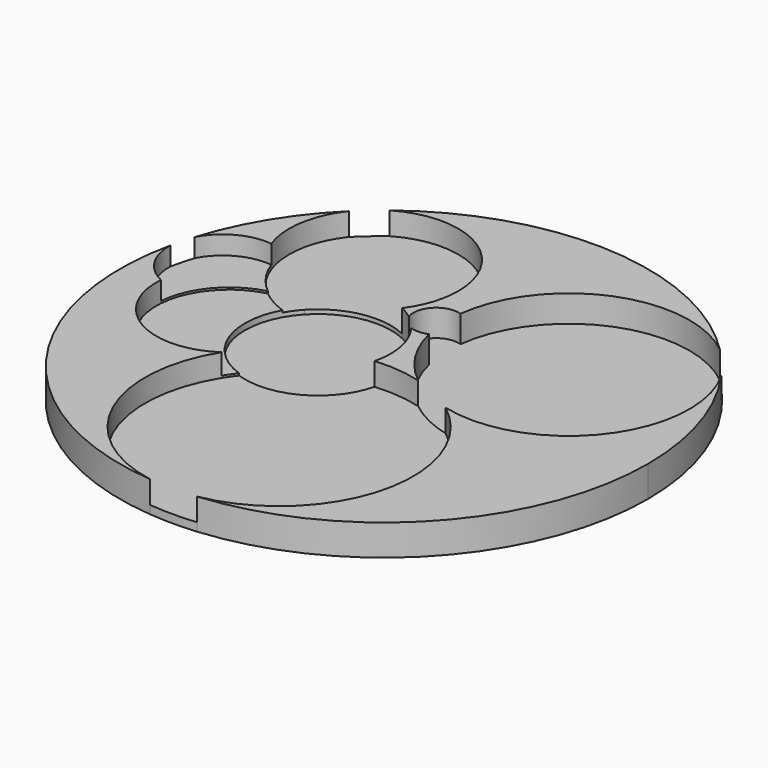
from build123d import *

# Parameters (mm, degrees)
F1_DEPTH = 1.5
F2_DEPTH = 1.1
F3_DEPTH = 1.3
F4_DEPTH = 1
F5_DEPTH = 0.9
F6_DEPTH = 1.3
F7_DEPTH = 1.3
F8_DEPTH = 1.1


with BuildPart() as f1:
    # F0 (on Top) → F1 (new body)
    with BuildSketch(Plane.XY):
        with BuildLine():
            ThreePointArc((1.1413139167, -12.749015748), (9.4458673009, -8.6380316585), (12.8, 0))
            ThreePointArc((12.8, 0), (12.2037895541, 3.8610258375), (10.470699919, 7.3623666851))
            ThreePointArc((10.470699919, 7.3623666851), (10.0212563072, 0.9384212672), (3.9401496855, -1.1803558676))
            ThreePointArc((3.9401496855, -1.1803558676), (6.3177362198, -7.8784662435), (1.1413139167, -12.749015748))
        make_face()
        with BuildLine():
            ThreePointArc((3.9401496855, -1.1803558676), (10.0212563072, 0.9384212672), (10.470699919, 7.3623666851))
            ThreePointArc((10.470699919, 7.3623666851), (9.8213681495, 8.2085764705), (9.1038369322, 8.9977860117))
            ThreePointArc((9.1038369322, 8.9977860117), (3.2034297018, 9.9238080984), (-0.4347578085, 5.1871516796))
            ThreePointArc((-0.4347578085, 5.1871516796), (0.1140807918, 4.7873856476), (0.3236429235, 4.1415370565))
            ThreePointArc((0.3236429235, 4.1415370565), (0.1493131035, 3.5472856637), (-0.3184201999, 3.1413901588))
            ThreePointArc((-0.3184201999, 3.1413901588), (0.4342128527, 1.3569660974), (1.7281912806, -0.0839522107))
            ThreePointArc((1.7281912806, -0.0839522107), (2.8867018502, -0.5261737296), (3.9401496855, -1.1803558676))
        make_face()
        with BuildLine():
            ThreePointArc((-1.1413139167, -12.749015748), (0, -12.8), (1.1413139167, -12.749015748))
            ThreePointArc((1.1413139167, -12.749015748), (6.3177362198, -7.8784662435), (3.9401496855, -1.1803558676))
            ThreePointArc((3.9401496855, -1.1803558676), (2.7756748559, -0.7501670477), (1.7281912806, -0.0839522107))
            ThreePointArc((1.7281912806, -0.0839522107), (0.596280043, 0.1225922249), (-0.554315346, 0.1263210619))
            ThreePointArc((-0.554315346, 0.1263210619), (-2.2047100942, -2.0697503993), (-4.9291383896, -2.4219196064))
            ThreePointArc((-4.9291383896, -2.4219196064), (-5.2141366822, -2.6925550862), (-5.5274388721, -2.9298509512))
            ThreePointArc((-5.5274388721, -2.9298509512), (-5.9348180483, -9.0010252232), (-1.1413139167, -12.749015748))
        make_face()
        with BuildLine():
            ThreePointArc((-0.4347578085, 5.1871516796), (3.2034297018, 9.9238080984), (9.1038369322, 8.9977860117))
            ThreePointArc((9.1038369322, 8.9977860117), (0.8515670805, 12.7716417702), (-7.8286793929, 10.1267852235))
            ThreePointArc((-7.8286793929, 10.1267852235), (-3.7190007865, 10.1436555147), (-1.6592760481, 6.5873545071))
            ThreePointArc((-1.6592760481, 6.5873545071), (-1.8611994375, 5.316528501), (-2.4470803104, 4.1708778581))
            ThreePointArc((-2.4470803104, 4.1708778581), (-2.1205912314, 3.9914565549), (-1.8147879972, 3.7786855401))
            ThreePointArc((-1.8147879972, 3.7786855401), (-1.5620655496, 4.9113826225), (-0.4347578085, 5.1871516796))
        make_face()
        with BuildLine():
            ThreePointArc((1.7281912806, -0.0839522107), (2.7756748559, -0.7501670477), (3.9401496855, -1.1803558676))
            ThreePointArc((3.9401496855, -1.1803558676), (2.8867018502, -0.5261737296), (1.7281912806, -0.0839522107))
        make_face()
        with BuildLine():
            ThreePointArc((-12.5092777133, 2.7125580349), (-10.3126004927, -7.5822339107), (-1.1413139167, -12.749015748))
            ThreePointArc((-1.1413139167, -12.749015748), (-5.9348180483, -9.0010252232), (-5.5274388721, -2.9298509512))
            ThreePointArc((-5.5274388721, -2.9298509512), (-9.2745377761, -3.053856526), (-11.0221912783, 0.2630448617))
            ThreePointArc((-11.0221912783, 0.2630448617), (-12.1336526301, 1.2644403034), (-12.5092777133, 2.7125580349))
        make_face()
        with BuildLine():
            ThreePointArc((-1.6592760481, 6.5873545071), (-3.7190007865, 10.1436555147), (-7.8286793929, 10.1267852235))
            ThreePointArc((-7.8286793929, 10.1267852235), (-8.4249981047, 9.6363585932), (-8.9906633635, 9.1108711046))
            ThreePointArc((-8.9906633635, 9.1108711046), (-9.8078763851, 7.234529376), (-9.6163122558, 5.1969330987))
            ThreePointArc((-9.6163122558, 5.1969330987), (-8.3134717361, 4.6648999744), (-7.4786994453, 3.5319357704))
            ThreePointArc((-7.4786994453, 3.5319357704), (-7.0171820767, 3.4988442167), (-6.5639507121, 3.4057063483))
            ThreePointArc((-6.5639507121, 3.4057063483), (-4.6309358982, 4.4630943822), (-2.4470803104, 4.1708778581))
            ThreePointArc((-2.4470803104, 4.1708778581), (-1.8611994375, 5.316528501), (-1.6592760481, 6.5873545071))
        make_face()
        with BuildLine():
            ThreePointArc((0.3236429235, 4.1415370565), (0.1140807918, 4.7873856476), (-0.4347578085, 5.1871516796))
            ThreePointArc((-0.4347578085, 5.1871516796), (-0.4668571228, 4.1591375853), (-0.3184201999, 3.1413901588))
            ThreePointArc((-0.3184201999, 3.1413901588), (0.1493131035, 3.5472856637), (0.3236429235, 4.1415370565))
        make_face()
        with BuildLine():
            ThreePointArc((-0.3184201999, 3.1413901588), (-0.4668571228, 4.1591375853), (-0.4347578085, 5.1871516796))
            ThreePointArc((-0.4347578085, 5.1871516796), (-1.5620655496, 4.9113826225), (-1.8147879972, 3.7786855401))
            ThreePointArc((-1.8147879972, 3.7786855401), (-1.4632990979, 3.4659314694), (-1.1564367138, 3.1092873438))
            ThreePointArc((-1.1564367138, 3.1092873438), (-0.7342490593, 3.0423432998), (-0.3184201999, 3.1413901588))
        make_face()
        with BuildLine():
            ThreePointArc((-0.554315346, 0.1263210619), (0.596280043, 0.1225922249), (1.7281912806, -0.0839522107))
            ThreePointArc((1.7281912806, -0.0839522107), (0.4342128527, 1.3569660974), (-0.3184201999, 3.1413901588))
            ThreePointArc((-0.3184201999, 3.1413901588), (-0.7342490593, 3.0423432998), (-1.1564367138, 3.1092873438))
            ThreePointArc((-1.1564367138, 3.1092873438), (-0.6299288982, 2.1052191407), (-0.4482007155, 0.9861399191))
            ThreePointArc((-0.4482007155, 0.9861399191), (-0.4748296274, 0.5529688265), (-0.554315346, 0.1263210619))
        make_face()
        with BuildLine():
            ThreePointArc((-12.2201512567, 3.8089241608), (-12.3768602224, 3.2639440918), (-12.5092777133, 2.7125580349))
            ThreePointArc((-12.5092777133, 2.7125580349), (-12.1336526301, 1.2644403034), (-11.0221912783, 0.2630448617))
            ThreePointArc((-11.0221912783, 0.2630448617), (-10.204575831, 2.2716279569), (-8.3673749649, 3.4238406316))
            ThreePointArc((-8.3673749649, 3.4238406316), (-9.1112094109, 4.2263075504), (-9.6163122558, 5.1969330987))
            ThreePointArc((-9.6163122558, 5.1969330987), (-11.1342032079, 4.90808084), (-12.2201512567, 3.8089241608))
        make_face()
        with BuildLine():
            ThreePointArc((-11.0221912783, 0.2630448617), (-9.2745377761, -3.053856526), (-5.5274388721, -2.9298509512))
            ThreePointArc((-5.5274388721, -2.9298509512), (-5.3367748168, -2.6393619746), (-5.1308600113, -2.3594767831))
            ThreePointArc((-5.1308600113, -2.3594767831), (-7.2860930404, -0.2817879048), (-7.075700244, 2.704439708))
            ThreePointArc((-7.075700244, 2.704439708), (-7.1973059974, 2.7478141876), (-7.3174857567, 2.7949960715))
            ThreePointArc((-7.3174857567, 2.7949960715), (-8.4441033358, 0.4671377871), (-11.0221912783, 0.2630448617))
        make_face()
        with BuildLine():
            ThreePointArc((-5.1308600113, -2.3594767831), (-5.3367748168, -2.6393619746), (-5.5274388721, -2.9298509512))
            ThreePointArc((-5.5274388721, -2.9298509512), (-5.2141366822, -2.6925550862), (-4.9291383896, -2.4219196064))
            ThreePointArc((-4.9291383896, -2.4219196064), (-5.0304653636, -2.3922041354), (-5.1308600113, -2.3594767831))
        make_face()
        with BuildLine():
            ThreePointArc((-9.6163122558, 5.1969330987), (-9.8078763851, 7.234529376), (-8.9906633635, 9.1108711046))
            ThreePointArc((-8.9906633635, 9.1108711046), (-10.931711877, 6.6586541762), (-12.2201512567, 3.8089241608))
            ThreePointArc((-12.2201512567, 3.8089241608), (-11.1342032079, 4.90808084), (-9.6163122558, 5.1969330987))
        make_face()
        with BuildLine():
            ThreePointArc((-1.1564367138, 3.1092873438), (-1.5606188549, 3.3702177563), (-1.8147879972, 3.7786855401))
            ThreePointArc((-1.8147879972, 3.7786855401), (-2.1205912314, 3.9914565549), (-2.4470803104, 4.1708778581))
            ThreePointArc((-2.4470803104, 4.1708778581), (-3.5931195136, 3.1062963536), (-5.0544484876, 2.5483920029))
            ThreePointArc((-5.0544484876, 2.5483920029), (-4.2509453728, 1.3851599291), (-3.968, 0))
            ThreePointArc((-3.968, 0), (-4.048144568, -0.7481430857), (-4.2849411533, -1.4623339606))
            ThreePointArc((-4.2849411533, -1.4623339606), (-2.5466756884, -0.3696619712), (-0.554315346, 0.1263210619))
            ThreePointArc((-0.554315346, 0.1263210619), (-0.4748296274, 0.5529688265), (-0.4482007155, 0.9861399191))
            ThreePointArc((-0.4482007155, 0.9861399191), (-0.6299288982, 2.1052191407), (-1.1564367138, 3.1092873438))
        make_face()
        with BuildLine():
            ThreePointArc((-1.1564367138, 3.1092873438), (-1.4632990979, 3.4659314694), (-1.8147879972, 3.7786855401))
            ThreePointArc((-1.8147879972, 3.7786855401), (-1.5606188549, 3.3702177563), (-1.1564367138, 3.1092873438))
        make_face()
        with BuildLine():
            ThreePointArc((-4.9291383896, -2.4219196064), (-2.2047100942, -2.0697503993), (-0.554315346, 0.1263210619))
            ThreePointArc((-0.554315346, 0.1263210619), (-2.5466756884, -0.3696619712), (-4.2849411533, -1.4623339606))
            ThreePointArc((-4.2849411533, -1.4623339606), (-4.5675232248, -1.9686553693), (-4.9291383896, -2.4219196064))
        make_face()
        with BuildLine():
            ThreePointArc((-8.3673749649, 3.4238406316), (-10.204575831, 2.2716279569), (-11.0221912783, 0.2630448617))
            ThreePointArc((-11.0221912783, 0.2630448617), (-8.4441033358, 0.4671377871), (-7.3174857567, 2.7949960715))
            ThreePointArc((-7.3174857567, 2.7949960715), (-7.8660255018, 3.0700250173), (-8.3673749649, 3.4238406316))
        make_face()
        with BuildLine():
            ThreePointArc((-7.075700244, 2.704439708), (-7.2860930404, -0.2817879048), (-5.1308600113, -2.3594767831))
            ThreePointArc((-5.1308600113, -2.3594767831), (-4.7292223678, -1.8908009917), (-4.2849411533, -1.4623339606))
            ThreePointArc((-4.2849411533, -1.4623339606), (-4.048144568, -0.7481430857), (-3.968, 0))
            ThreePointArc((-3.968, 0), (-4.2509453728, 1.3851599291), (-5.0544484876, 2.5483920029))
            ThreePointArc((-5.0544484876, 2.5483920029), (-6.0748712519, 2.4995189346), (-7.075700244, 2.704439708))
        make_face()
        with BuildLine():
            ThreePointArc((-4.2849411533, -1.4623339606), (-4.7292223678, -1.8908009917), (-5.1308600113, -2.3594767831))
            ThreePointArc((-5.1308600113, -2.3594767831), (-5.0304653636, -2.3922041354), (-4.9291383896, -2.4219196064))
            ThreePointArc((-4.9291383896, -2.4219196064), (-4.5675232248, -1.9686553693), (-4.2849411533, -1.4623339606))
        make_face()
        with BuildLine():
            ThreePointArc((-7.4786994453, 3.5319357704), (-8.3134717361, 4.6648999744), (-9.6163122558, 5.1969330987))
            ThreePointArc((-9.6163122558, 5.1969330987), (-9.1112094109, 4.2263075504), (-8.3673749649, 3.4238406316))
            ThreePointArc((-8.3673749649, 3.4238406316), (-7.9264758102, 3.5061577807), (-7.4786994453, 3.5319357704))
        make_face()
        with BuildLine():
            ThreePointArc((-5.0544484876, 2.5483920029), (-3.5931195136, 3.1062963536), (-2.4470803104, 4.1708778581))
            ThreePointArc((-2.4470803104, 4.1708778581), (-4.6309358982, 4.4630943822), (-6.5639507121, 3.4057063483))
            ThreePointArc((-6.5639507121, 3.4057063483), (-5.7557084634, 3.0712328201), (-5.0544484876, 2.5483920029))
        make_face()
        with BuildLine():
            ThreePointArc((-7.4786994453, 3.5319357704), (-7.9264758102, 3.5061577807), (-8.3673749649, 3.4238406316))
            ThreePointArc((-8.3673749649, 3.4238406316), (-7.8660255018, 3.0700250173), (-7.3174857567, 2.7949960715))
            ThreePointArc((-7.3174857567, 2.7949960715), (-7.3712234042, 3.1693438542), (-7.4786994453, 3.5319357704))
        make_face()
        with BuildLine():
            ThreePointArc((-7.4786994453, 3.5319357704), (-7.3712234042, 3.1693438542), (-7.3174857567, 2.7949960715))
            ThreePointArc((-7.3174857567, 2.7949960715), (-7.1973059974, 2.7478141876), (-7.075700244, 2.704439708))
            ThreePointArc((-7.075700244, 2.704439708), (-6.8414254387, 3.0708356057), (-6.5639507121, 3.4057063483))
            ThreePointArc((-6.5639507121, 3.4057063483), (-7.0171820767, 3.4988442167), (-7.4786994453, 3.5319357704))
        make_face()
        with BuildLine():
            ThreePointArc((-6.5639507121, 3.4057063483), (-6.8414254387, 3.0708356057), (-7.075700244, 2.704439708))
            ThreePointArc((-7.075700244, 2.704439708), (-6.0748712519, 2.4995189346), (-5.0544484876, 2.5483920029))
            ThreePointArc((-5.0544484876, 2.5483920029), (-5.7557084634, 3.0712328201), (-6.5639507121, 3.4057063483))
        make_face()
    extrude(amount=-F1_DEPTH)

    # F0 (on Top) → F2 (cut)
    with BuildSketch(Plane.XY):
        with BuildLine():
            ThreePointArc((-1.1413139167, -12.749015748), (0, -12.85), (1.1413139167, -12.749015748))
            ThreePointArc((1.1413139167, -12.749015748), (0, -12.8), (-1.1413139167, -12.749015748))
        make_face()
        with BuildLine():
            ThreePointArc((-1.1413139167, -12.749015748), (0, -12.8), (1.1413139167, -12.749015748))
            ThreePointArc((1.1413139167, -12.749015748), (6.3177362198, -7.8784662435), (3.9401496855, -1.1803558676))
            ThreePointArc((3.9401496855, -1.1803558676), (2.7756748559, -0.7501670477), (1.7281912806, -0.0839522107))
            ThreePointArc((1.7281912806, -0.0839522107), (0.596280043, 0.1225922249), (-0.554315346, 0.1263210619))
            ThreePointArc((-0.554315346, 0.1263210619), (-2.2047100942, -2.0697503993), (-4.9291383896, -2.4219196064))
            ThreePointArc((-4.9291383896, -2.4219196064), (-5.2141366822, -2.6925550862), (-5.5274388721, -2.9298509512))
            ThreePointArc((-5.5274388721, -2.9298509512), (-5.9348180483, -9.0010252232), (-1.1413139167, -12.749015748))
        make_face()
        with BuildLine():
            ThreePointArc((1.7281912806, -0.0839522107), (2.7756748559, -0.7501670477), (3.9401496855, -1.1803558676))
            ThreePointArc((3.9401496855, -1.1803558676), (2.8867018502, -0.5261737296), (1.7281912806, -0.0839522107))
        make_face()
        with BuildLine():
            ThreePointArc((-4.9291383896, -2.4219196064), (-2.2047100942, -2.0697503993), (-0.554315346, 0.1263210619))
            ThreePointArc((-0.554315346, 0.1263210619), (-2.5466756884, -0.3696619712), (-4.2849411533, -1.4623339606))
            ThreePointArc((-4.2849411533, -1.4623339606), (-4.5675232248, -1.9686553693), (-4.9291383896, -2.4219196064))
        make_face()
        with BuildLine():
            ThreePointArc((-4.2849411533, -1.4623339606), (-4.7292223678, -1.8908009917), (-5.1308600113, -2.3594767831))
            ThreePointArc((-5.1308600113, -2.3594767831), (-5.0304653636, -2.3922041354), (-4.9291383896, -2.4219196064))
            ThreePointArc((-4.9291383896, -2.4219196064), (-4.5675232248, -1.9686553693), (-4.2849411533, -1.4623339606))
        make_face()
        with BuildLine():
            ThreePointArc((-5.1308600113, -2.3594767831), (-5.3367748168, -2.6393619746), (-5.5274388721, -2.9298509512))
            ThreePointArc((-5.5274388721, -2.9298509512), (-5.2141366822, -2.6925550862), (-4.9291383896, -2.4219196064))
            ThreePointArc((-4.9291383896, -2.4219196064), (-5.0304653636, -2.3922041354), (-5.1308600113, -2.3594767831))
        make_face()
    extrude(amount=-F2_DEPTH, mode=Mode.SUBTRACT)

    # F0 (on Top) → F3 (cut)
    with BuildSketch(Plane.XY):
        with BuildLine():
            ThreePointArc((-7.075700244, 2.704439708), (-7.2860930404, -0.2817879048), (-5.1308600113, -2.3594767831))
            ThreePointArc((-5.1308600113, -2.3594767831), (-4.7292223678, -1.8908009917), (-4.2849411533, -1.4623339606))
            ThreePointArc((-4.2849411533, -1.4623339606), (-4.048144568, -0.7481430857), (-3.968, 0))
            ThreePointArc((-3.968, 0), (-4.2509453728, 1.3851599291), (-5.0544484876, 2.5483920029))
            ThreePointArc((-5.0544484876, 2.5483920029), (-6.0748712519, 2.4995189346), (-7.075700244, 2.704439708))
        make_face()
        with BuildLine():
            ThreePointArc((-1.1564367138, 3.1092873438), (-1.5606188549, 3.3702177563), (-1.8147879972, 3.7786855401))
            ThreePointArc((-1.8147879972, 3.7786855401), (-2.1205912314, 3.9914565549), (-2.4470803104, 4.1708778581))
            ThreePointArc((-2.4470803104, 4.1708778581), (-3.5931195136, 3.1062963536), (-5.0544484876, 2.5483920029))
            ThreePointArc((-5.0544484876, 2.5483920029), (-4.2509453728, 1.3851599291), (-3.968, 0))
            ThreePointArc((-3.968, 0), (-4.048144568, -0.7481430857), (-4.2849411533, -1.4623339606))
            ThreePointArc((-4.2849411533, -1.4623339606), (-2.5466756884, -0.3696619712), (-0.554315346, 0.1263210619))
            ThreePointArc((-0.554315346, 0.1263210619), (-0.4748296274, 0.5529688265), (-0.4482007155, 0.9861399191))
            ThreePointArc((-0.4482007155, 0.9861399191), (-0.6299288982, 2.1052191407), (-1.1564367138, 3.1092873438))
        make_face()
        with BuildLine():
            ThreePointArc((-5.0544484876, 2.5483920029), (-3.5931195136, 3.1062963536), (-2.4470803104, 4.1708778581))
            ThreePointArc((-2.4470803104, 4.1708778581), (-4.6309358982, 4.4630943822), (-6.5639507121, 3.4057063483))
            ThreePointArc((-6.5639507121, 3.4057063483), (-5.7557084634, 3.0712328201), (-5.0544484876, 2.5483920029))
        make_face()
        with BuildLine():
            ThreePointArc((-6.5639507121, 3.4057063483), (-6.8414254387, 3.0708356057), (-7.075700244, 2.704439708))
            ThreePointArc((-7.075700244, 2.704439708), (-6.0748712519, 2.4995189346), (-5.0544484876, 2.5483920029))
            ThreePointArc((-5.0544484876, 2.5483920029), (-5.7557084634, 3.0712328201), (-6.5639507121, 3.4057063483))
        make_face()
        with BuildLine():
            ThreePointArc((-4.9291383896, -2.4219196064), (-2.2047100942, -2.0697503993), (-0.554315346, 0.1263210619))
            ThreePointArc((-0.554315346, 0.1263210619), (-2.5466756884, -0.3696619712), (-4.2849411533, -1.4623339606))
            ThreePointArc((-4.2849411533, -1.4623339606), (-4.5675232248, -1.9686553693), (-4.9291383896, -2.4219196064))
        make_face()
        with BuildLine():
            ThreePointArc((-4.2849411533, -1.4623339606), (-4.7292223678, -1.8908009917), (-5.1308600113, -2.3594767831))
            ThreePointArc((-5.1308600113, -2.3594767831), (-5.0304653636, -2.3922041354), (-4.9291383896, -2.4219196064))
            ThreePointArc((-4.9291383896, -2.4219196064), (-4.5675232248, -1.9686553693), (-4.2849411533, -1.4623339606))
        make_face()
        with BuildLine():
            ThreePointArc((-1.1564367138, 3.1092873438), (-1.4632990979, 3.4659314694), (-1.8147879972, 3.7786855401))
            ThreePointArc((-1.8147879972, 3.7786855401), (-1.5606188549, 3.3702177563), (-1.1564367138, 3.1092873438))
        make_face()
    extrude(amount=-F3_DEPTH, mode=Mode.SUBTRACT)

    # F0 (on Top) → F4 (cut)
    with BuildSketch(Plane.XY):
        with BuildLine():
            ThreePointArc((-11.0221912783, 0.2630448617), (-9.2745377761, -3.053856526), (-5.5274388721, -2.9298509512))
            ThreePointArc((-5.5274388721, -2.9298509512), (-5.3367748168, -2.6393619746), (-5.1308600113, -2.3594767831))
            ThreePointArc((-5.1308600113, -2.3594767831), (-7.2860930404, -0.2817879048), (-7.075700244, 2.704439708))
            ThreePointArc((-7.075700244, 2.704439708), (-7.1973059974, 2.7478141876), (-7.3174857567, 2.7949960715))
            ThreePointArc((-7.3174857567, 2.7949960715), (-8.4441033358, 0.4671377871), (-11.0221912783, 0.2630448617))
        make_face()
        with BuildLine():
            ThreePointArc((-8.3673749649, 3.4238406316), (-10.204575831, 2.2716279569), (-11.0221912783, 0.2630448617))
            ThreePointArc((-11.0221912783, 0.2630448617), (-8.4441033358, 0.4671377871), (-7.3174857567, 2.7949960715))
            ThreePointArc((-7.3174857567, 2.7949960715), (-7.8660255018, 3.0700250173), (-8.3673749649, 3.4238406316))
        make_face()
        with BuildLine():
            ThreePointArc((-7.4786994453, 3.5319357704), (-7.9264758102, 3.5061577807), (-8.3673749649, 3.4238406316))
            ThreePointArc((-8.3673749649, 3.4238406316), (-7.8660255018, 3.0700250173), (-7.3174857567, 2.7949960715))
            ThreePointArc((-7.3174857567, 2.7949960715), (-7.3712234042, 3.1693438542), (-7.4786994453, 3.5319357704))
        make_face()
        with BuildLine():
            ThreePointArc((-7.4786994453, 3.5319357704), (-7.3712234042, 3.1693438542), (-7.3174857567, 2.7949960715))
            ThreePointArc((-7.3174857567, 2.7949960715), (-7.1973059974, 2.7478141876), (-7.075700244, 2.704439708))
            ThreePointArc((-7.075700244, 2.704439708), (-6.8414254387, 3.0708356057), (-6.5639507121, 3.4057063483))
            ThreePointArc((-6.5639507121, 3.4057063483), (-7.0171820767, 3.4988442167), (-7.4786994453, 3.5319357704))
        make_face()
    extrude(amount=-F4_DEPTH, mode=Mode.SUBTRACT)

    # F0 (on Top) → F5 (cut)
    with BuildSketch(Plane.XY):
        with BuildLine():
            ThreePointArc((-12.2201512567, 3.8089241608), (-12.3768602224, 3.2639440918), (-12.5092777133, 2.7125580349))
            ThreePointArc((-12.5092777133, 2.7125580349), (-12.1336526301, 1.2644403034), (-11.0221912783, 0.2630448617))
            ThreePointArc((-11.0221912783, 0.2630448617), (-10.204575831, 2.2716279569), (-8.3673749649, 3.4238406316))
            ThreePointArc((-8.3673749649, 3.4238406316), (-9.1112094109, 4.2263075504), (-9.6163122558, 5.1969330987))
            ThreePointArc((-9.6163122558, 5.1969330987), (-11.1342032079, 4.90808084), (-12.2201512567, 3.8089241608))
        make_face()
        with BuildLine():
            ThreePointArc((-7.4786994453, 3.5319357704), (-8.3134717361, 4.6648999744), (-9.6163122558, 5.1969330987))
            ThreePointArc((-9.6163122558, 5.1969330987), (-9.1112094109, 4.2263075504), (-8.3673749649, 3.4238406316))
            ThreePointArc((-8.3673749649, 3.4238406316), (-7.9264758102, 3.5061577807), (-7.4786994453, 3.5319357704))
        make_face()
    extrude(amount=-F5_DEPTH, mode=Mode.SUBTRACT)

    # F0 (on Top) → F6 (cut)
    with BuildSketch(Plane.XY):
        with BuildLine():
            ThreePointArc((3.9401496855, -1.1803558676), (10.0212563072, 0.9384212672), (10.470699919, 7.3623666851))
            ThreePointArc((10.470699919, 7.3623666851), (9.8213681495, 8.2085764705), (9.1038369322, 8.9977860117))
            ThreePointArc((9.1038369322, 8.9977860117), (3.2034297018, 9.9238080984), (-0.4347578085, 5.1871516796))
            ThreePointArc((-0.4347578085, 5.1871516796), (0.1140807918, 4.7873856476), (0.3236429235, 4.1415370565))
            ThreePointArc((0.3236429235, 4.1415370565), (0.1493131035, 3.5472856637), (-0.3184201999, 3.1413901588))
            ThreePointArc((-0.3184201999, 3.1413901588), (0.4342128527, 1.3569660974), (1.7281912806, -0.0839522107))
            ThreePointArc((1.7281912806, -0.0839522107), (2.8867018502, -0.5261737296), (3.9401496855, -1.1803558676))
        make_face()
        with BuildLine():
            ThreePointArc((0.3236429235, 4.1415370565), (0.1140807918, 4.7873856476), (-0.4347578085, 5.1871516796))
            ThreePointArc((-0.4347578085, 5.1871516796), (-0.4668571228, 4.1591375853), (-0.3184201999, 3.1413901588))
            ThreePointArc((-0.3184201999, 3.1413901588), (0.1493131035, 3.5472856637), (0.3236429235, 4.1415370565))
        make_face()
        with BuildLine():
            ThreePointArc((1.7281912806, -0.0839522107), (2.7756748559, -0.7501670477), (3.9401496855, -1.1803558676))
            ThreePointArc((3.9401496855, -1.1803558676), (2.8867018502, -0.5261737296), (1.7281912806, -0.0839522107))
        make_face()
        with BuildLine():
            ThreePointArc((9.1038369322, 8.9977860117), (9.8213681495, 8.2085764705), (10.470699919, 7.3623666851))
            ThreePointArc((10.470699919, 7.3623666851), (9.8623786831, 8.2428525608), (9.1038369322, 8.9977860117))
        make_face()
    extrude(amount=-F6_DEPTH, mode=Mode.SUBTRACT)

    # F0 (on Top) → F7 (cut)
    with BuildSketch(Plane.XY):
        with BuildLine():
            ThreePointArc((-0.3184201999, 3.1413901588), (-0.4668571228, 4.1591375853), (-0.4347578085, 5.1871516796))
            ThreePointArc((-0.4347578085, 5.1871516796), (-1.5620655496, 4.9113826225), (-1.8147879972, 3.7786855401))
            ThreePointArc((-1.8147879972, 3.7786855401), (-1.4632990979, 3.4659314694), (-1.1564367138, 3.1092873438))
            ThreePointArc((-1.1564367138, 3.1092873438), (-0.7342490593, 3.0423432998), (-0.3184201999, 3.1413901588))
        make_face()
        with BuildLine():
            ThreePointArc((0.3236429235, 4.1415370565), (0.1140807918, 4.7873856476), (-0.4347578085, 5.1871516796))
            ThreePointArc((-0.4347578085, 5.1871516796), (-0.4668571228, 4.1591375853), (-0.3184201999, 3.1413901588))
            ThreePointArc((-0.3184201999, 3.1413901588), (0.1493131035, 3.5472856637), (0.3236429235, 4.1415370565))
        make_face()
        with BuildLine():
            ThreePointArc((-1.1564367138, 3.1092873438), (-1.4632990979, 3.4659314694), (-1.8147879972, 3.7786855401))
            ThreePointArc((-1.8147879972, 3.7786855401), (-1.5606188549, 3.3702177563), (-1.1564367138, 3.1092873438))
        make_face()
    extrude(amount=-F7_DEPTH, mode=Mode.SUBTRACT)

    # F0 (on Top) → F8 (cut)
    with BuildSketch(Plane.XY):
        with BuildLine():
            ThreePointArc((-1.6592760481, 6.5873545071), (-3.7190007865, 10.1436555147), (-7.8286793929, 10.1267852235))
            ThreePointArc((-7.8286793929, 10.1267852235), (-8.4249981047, 9.6363585932), (-8.9906633635, 9.1108711046))
            ThreePointArc((-8.9906633635, 9.1108711046), (-9.8078763851, 7.234529376), (-9.6163122558, 5.1969330987))
            ThreePointArc((-9.6163122558, 5.1969330987), (-8.3134717361, 4.6648999744), (-7.4786994453, 3.5319357704))
            ThreePointArc((-7.4786994453, 3.5319357704), (-7.0171820767, 3.4988442167), (-6.5639507121, 3.4057063483))
            ThreePointArc((-6.5639507121, 3.4057063483), (-4.6309358982, 4.4630943822), (-2.4470803104, 4.1708778581))
            ThreePointArc((-2.4470803104, 4.1708778581), (-1.8611994375, 5.316528501), (-1.6592760481, 6.5873545071))
        make_face()
        with BuildLine():
            ThreePointArc((-7.4786994453, 3.5319357704), (-8.3134717361, 4.6648999744), (-9.6163122558, 5.1969330987))
            ThreePointArc((-9.6163122558, 5.1969330987), (-9.1112094109, 4.2263075504), (-8.3673749649, 3.4238406316))
            ThreePointArc((-8.3673749649, 3.4238406316), (-7.9264758102, 3.5061577807), (-7.4786994453, 3.5319357704))
        make_face()
        with BuildLine():
            ThreePointArc((-5.0544484876, 2.5483920029), (-3.5931195136, 3.1062963536), (-2.4470803104, 4.1708778581))
            ThreePointArc((-2.4470803104, 4.1708778581), (-4.6309358982, 4.4630943822), (-6.5639507121, 3.4057063483))
            ThreePointArc((-6.5639507121, 3.4057063483), (-5.7557084634, 3.0712328201), (-5.0544484876, 2.5483920029))
        make_face()
        with BuildLine():
            ThreePointArc((-6.5639507121, 3.4057063483), (-6.8414254387, 3.0708356057), (-7.075700244, 2.704439708))
            ThreePointArc((-7.075700244, 2.704439708), (-6.0748712519, 2.4995189346), (-5.0544484876, 2.5483920029))
            ThreePointArc((-5.0544484876, 2.5483920029), (-5.7557084634, 3.0712328201), (-6.5639507121, 3.4057063483))
        make_face()
        with BuildLine():
            ThreePointArc((-7.4786994453, 3.5319357704), (-7.9264758102, 3.5061577807), (-8.3673749649, 3.4238406316))
            ThreePointArc((-8.3673749649, 3.4238406316), (-7.8660255018, 3.0700250173), (-7.3174857567, 2.7949960715))
            ThreePointArc((-7.3174857567, 2.7949960715), (-7.3712234042, 3.1693438542), (-7.4786994453, 3.5319357704))
        make_face()
        with BuildLine():
            ThreePointArc((-7.4786994453, 3.5319357704), (-7.3712234042, 3.1693438542), (-7.3174857567, 2.7949960715))
            ThreePointArc((-7.3174857567, 2.7949960715), (-7.1973059974, 2.7478141876), (-7.075700244, 2.704439708))
            ThreePointArc((-7.075700244, 2.704439708), (-6.8414254387, 3.0708356057), (-6.5639507121, 3.4057063483))
            ThreePointArc((-6.5639507121, 3.4057063483), (-7.0171820767, 3.4988442167), (-7.4786994453, 3.5319357704))
        make_face()
    extrude(amount=-F8_DEPTH, mode=Mode.SUBTRACT)


solid = f1.part
